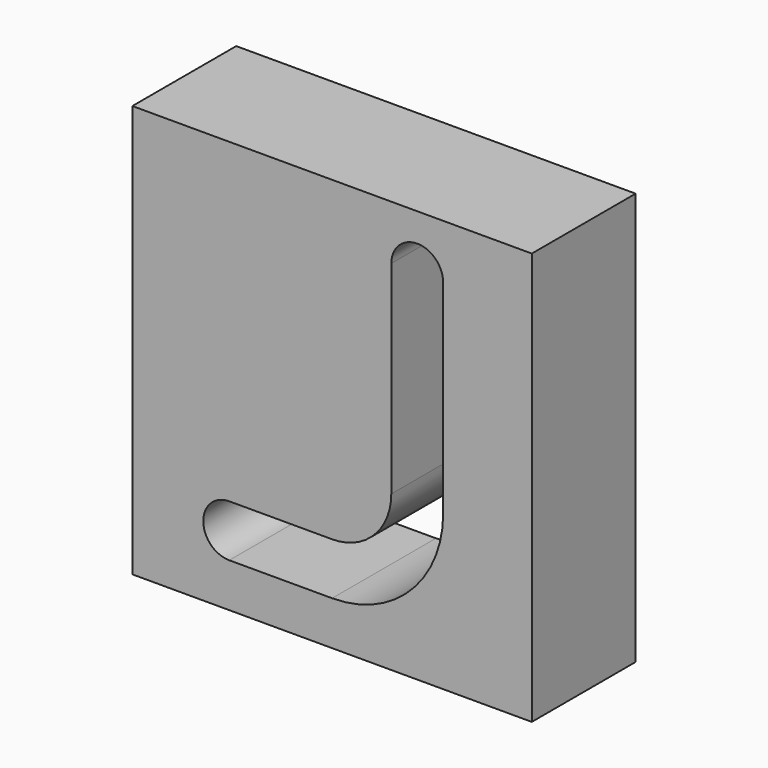
from build123d import *

# Parameters (mm, degrees)
F0_W     = 76.9356526434
F0_H     = 79.423185253
F1_DEPTH = 25


# Not quite as in the source:
# - ends of sketch curves that miss each other by under 0.0002 mm in the source are joined


with BuildPart() as f1:
    # F0 (on Front) → F1 (new body)
    with BuildSketch(Plane.XZ):
        Rectangle(F0_W, F0_H)
        with BuildLine():
            Line((11.4050824274, -9.8430258844), (11.4050824274, 29.2284450168))
            ThreePointArc((11.4050824274, 29.2284450168), (16.4050836887, 34.228446278), (21.4050849499, 29.2284450168))
            Line((21.4050849499, 29.2284450168), (21.4050824274, -9.8430258844))
            ThreePointArc((21.4050824274, -9.8430258844), (15.1356789363, -24.9787048207), (0, -31.2481083118))
            Line((0, -31.2481083118), (-19.8113770242, -31.2481083118))
            ThreePointArc((-19.8113770242, -31.2481083118), (-24.8113770242, -26.2481083118), (-19.8113770242, -21.2481083118))
            Line((-19.8113770242, -21.2481083118), (0, -21.2481083118))
            ThreePointArc((0, -21.2481083118), (8.0646111244, -17.9076370088), (11.4050824274, -9.8430258844))
        make_face(mode=Mode.SUBTRACT)
    extrude(amount=F1_DEPTH)


solid = f1.part
